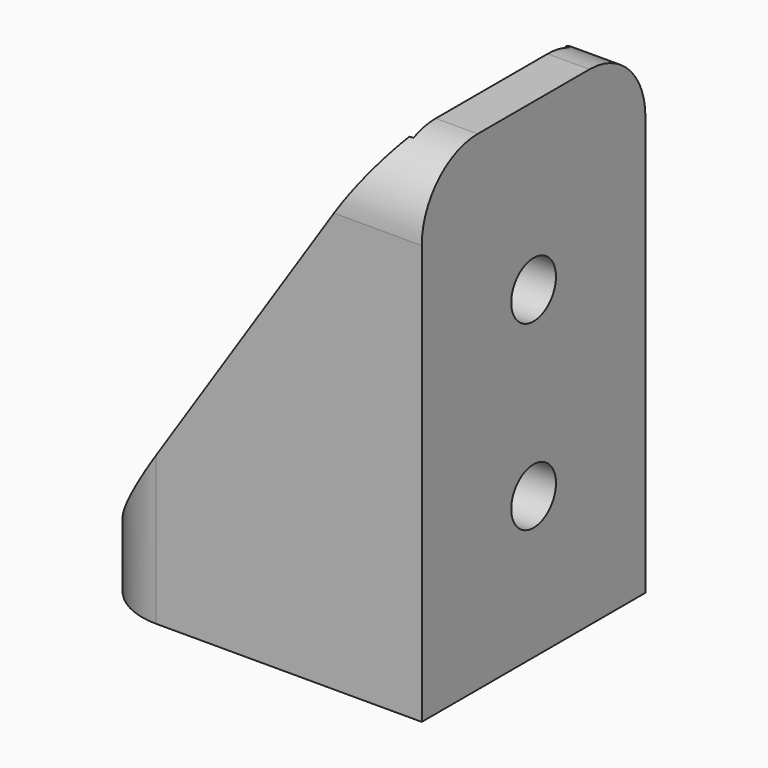
from build123d import *

# Parameters (mm, degrees)
F1_DEPTH        = 3
F2_W            = 3
F2_H            = 20
F3_DEPTH        = 32
F5_DEPTH        = 3
F8_D            = 4
F10_D           = 4
F10_CSINK_D     = 7
F10_CSINK_ANGLE = 90
F11_T1_DEPTH    = 28
F11_T3_DEPTH    = 28


# Not quite as in the source:
# - a fillet or chamfer that OpenCascade refuses, or shapes differently, is made with other operations: its cross-section is extruded or revolved along the edge and cut away or added


with BuildPart() as f1:
    # F0 (on Top) → F1 (new body)
    with BuildSketch(Plane.XY):
        Polygon((0, 10), (0, 0), (0, -10), (24, -10), (24, 0), (24, 10), align=None)
    extrude(amount=F1_DEPTH)

    # F2 (on face) → F3 (join)
    with BuildSketch(Plane.XY.offset(3)):
        with Locations((22.5, 0)):
            Rectangle(F2_W, F2_H)
    extrude(amount=F3_DEPTH)

    # F4 (on face) → F5 (join)
    with BuildSketch(Plane.XZ.offset(10)):
        Polygon((21, 3), (21, 35), (0, 3), align=None)
    extrude(amount=-F5_DEPTH)

    # F6: F1 across plane


with BuildPart() as f1_1:
    add(f1.part)
    add(f1.part.mirror(Plane.XZ))

    # F8 (through all)
    with Locations(Plane(origin=(21, 0, 0), x_dir=(0, -1, 0), z_dir=(-1, 0, 0))):
        with Locations((0, 10.16), (0, 23.16)):
            Hole(F8_D / 2)

    # F10 (through all)
    with Locations(Plane.XY.offset(3)):
        with Locations((10.5, 0)):
            CounterSinkHole(F10_D / 2, F10_CSINK_D / 2, counter_sink_angle=F10_CSINK_ANGLE)

    # F11: fillet of radius 5 on 4 edges, made by hand

    # F11_s2 → F11_t1 (cut)
    with BuildSketch(Plane.XY.offset(-12.5)):
        with BuildLine():
            ThreePointArc((0, -5), (1.4644660941, -8.5355339059), (5, -10))
            Line((5, -10), (0, -10))
            Line((0, -10), (0, -5))
        make_face()
        with BuildLine():
            ThreePointArc((0, 5), (1.4644660941, 8.5355339059), (5, 10))
            Line((5, 10), (0, 10))
            Line((0, 10), (0, 5))
        make_face()
    extrude(amount=F11_T1_DEPTH, mode=Mode.SUBTRACT)

    # F11_s4 → F11_t3 (cut)
    with BuildSketch(Plane.YZ.offset(8.5)):
        with BuildLine():
            ThreePointArc((-10, 30), (-8.5355339059, 33.5355339059), (-5, 35))
            Line((-5, 35), (-10, 35))
            Line((-10, 35), (-10, 30))
        make_face()
        with BuildLine():
            ThreePointArc((10, 30), (8.5355339059, 33.5355339059), (5, 35))
            Line((5, 35), (10, 35))
            Line((10, 35), (10, 30))
        make_face()
    extrude(amount=F11_T3_DEPTH, mode=Mode.SUBTRACT)


solid = f1_1.part
